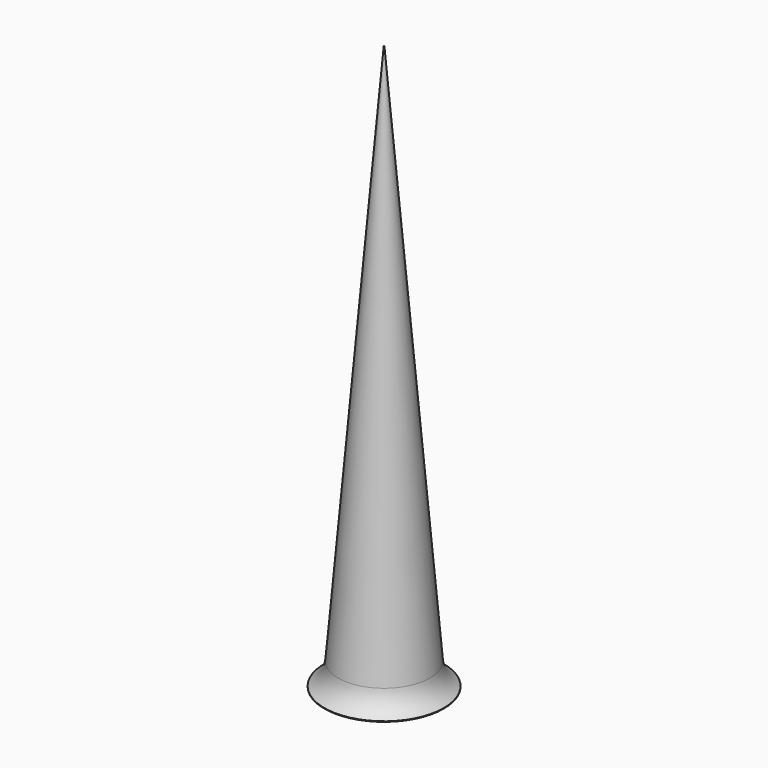
from build123d import *

# Parameters (mm, degrees)
F0_R     = 85
F2_R     = 0.5
F4_R     = 105.9677495378
F5_DEPTH = 1


# Not quite as in the source:
# - a fillet or chamfer that OpenCascade refuses, or shapes differently, is made with other operations: its cross-section is extruded or revolved along the edge and cut away or added


with BuildPart() as f3:
    # F0 (on Top) → F3 section 0
    with BuildSketch(Plane.XY):
        Circle(F0_R)
    # F2 (on offset) → F3 section 1
    with BuildSketch(Plane.XY.offset(1000)):
        Circle(F2_R)
    loft()

    # F4 (on Top) → F5 (join)
    with BuildSketch(Plane.XY):
        Circle(F4_R)
    extrude(amount=F5_DEPTH)

    # F6: fillet of radius 50 on 1 edges, made by hand

    # F6_s1 → F6_t2 (revolve)
    with BuildSketch(Plane.XZ):
        with BuildLine():
            ThreePointArc((105.9677495378, 1), (89.0977776327, 17.4521656578), (81.6365703283, 39.8039014399))
            Line((81.6365703283, 39.8039014399), (84.9155, 1))
            Line((84.9155, 1), (105.9677495378, 1))
        make_face()
    revolve(axis=Axis((0, 0, 1), (0, 0, 1)))


solid = f3.part
